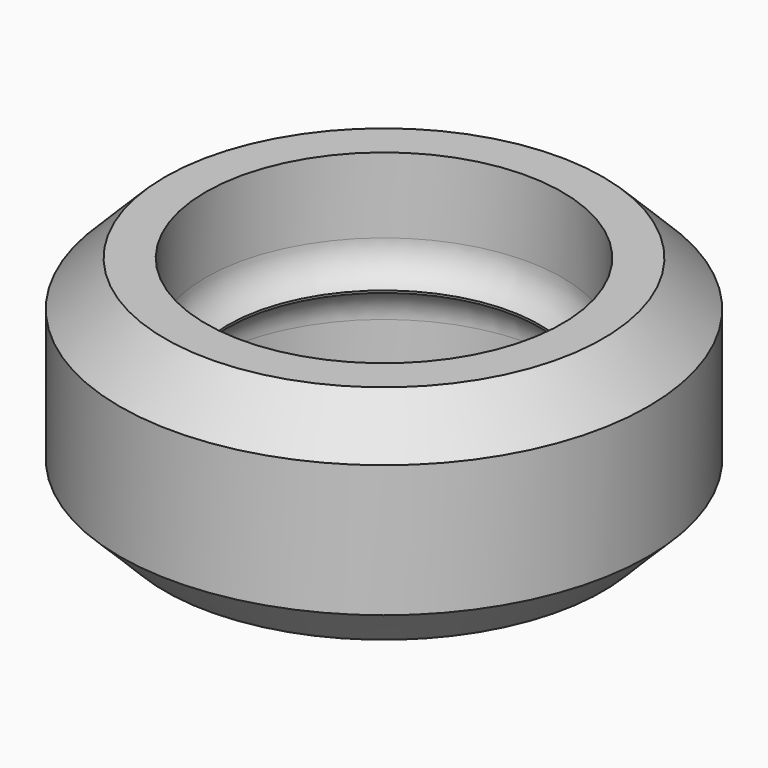
from build123d import *


# Not quite as in the source:
# - a fillet or chamfer that OpenCascade refuses, or shapes differently, is made with other operations: its cross-section is extruded or revolved along the edge and cut away or added


with BuildPart() as f1:
    # F0 (on Front) → F1 (revolve)
    with BuildSketch(Plane.XZ):
        Polygon((-7.1, 0.05), (-8.1, 0.05), (-8.1, 5.05), (-9.95, 5.05), (-12, 3), (-12, -3), (-9.95, -5.05), (-8.1, -5.05), (-8.1, -0.05), (-7.1, -0.05), align=None)
    revolve(axis=Axis((0, 0, 10.9107699245), (0, 0, -1)))

    # F2: fillet of radius 1.75 on 2 edges, made by hand

    # F2_s1 → F2_t2 (revolve)
    with BuildSketch(Plane.XZ):
        with BuildLine():
            ThreePointArc((-8.1, -1.6311388301), (-7.8290199458, -0.6957244834), (-7.1, -0.05))
            Line((-7.1, -0.05), (-7.115, -0.0183772234))
            ThreePointArc((-7.115, -0.0183772234), (-7.6, -0.015), (-8.1, -0.015))
            Line((-8.1, -0.015), (-8.135, -0.05))
            Line((-8.135, -0.05), (-8.135, -1.6311388301))
            Line((-8.135, -1.6311388301), (-8.1, -1.6311388301))
        make_face()
    revolve(axis=Axis((0, 0, -0.05), (0, 0, -1)))

    # F2_s3 → F2_t4 (revolve)
    with BuildSketch(Plane.XZ):
        with BuildLine():
            ThreePointArc((-7.1, 0.05), (-7.8290199458, 0.6957244834), (-8.1, 1.6311388301))
            Line((-8.1, 1.6311388301), (-8.135, 1.6311388301))
            Line((-8.135, 1.6311388301), (-8.135, 0.05))
            Line((-8.135, 0.05), (-8.1, 0.015))
            ThreePointArc((-8.1, 0.015), (-7.6, 0.015), (-7.115, 0.0183772234))
            Line((-7.115, 0.0183772234), (-7.1, 0.05))
        make_face()
    revolve(axis=Axis((0, 0, 0.05), (0, 0, -1)))


solid = f1.part
